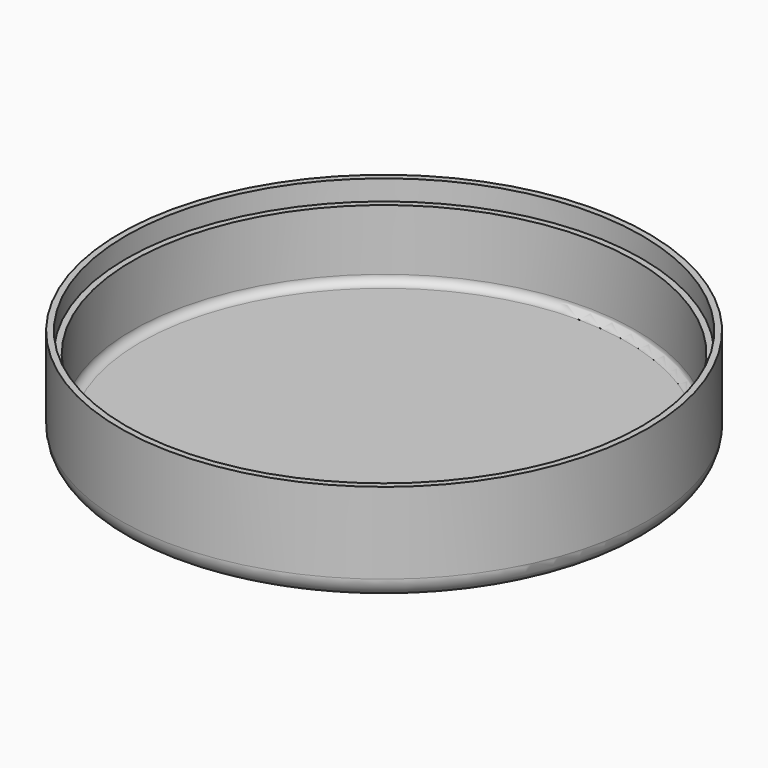
from build123d import *

# Parameters (mm, degrees)
F0_R     = 32.5
F1_DEPTH = 10
F2_R     = 2.5
F3_T     = -1.5
F4_R     = 32.5
F4_R_2   = 31.75
F5_DEPTH = 2.5


# Not quite as in the source:
# - a feature names something its author has since deleted; it is built from what else it names


with BuildPart() as f1:
    # F0 (on Top) → F1 (new body)
    with BuildSketch(Plane.XY):
        Circle(F0_R)
    extrude(amount=F1_DEPTH)

    # F2
    f2_edges = [f1.edges().sort_by_distance(p)[0] for p in [
        (-32.5, 0, 0),
    ]]
    fillet(f2_edges, radius=F2_R)

    # F3
    f3_openings = [f1.faces().sort_by_distance(p)[0] for p in [
        (0, 0, 10),
    ]]
    offset(amount=F3_T, openings=f3_openings)

    # F4 (on face) → F5 (join)
    with BuildSketch(Plane.XY.offset(10)):
        Circle(F4_R)
        Circle(F4_R_2, mode=Mode.SUBTRACT)
    extrude(amount=F5_DEPTH)


solid = f1.part
